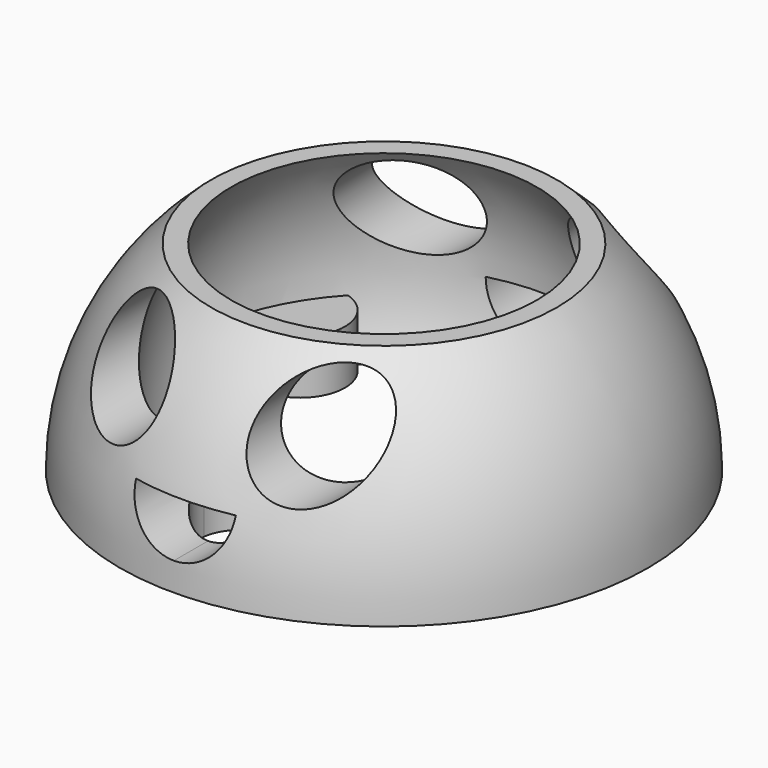
from build123d import *

# Parameters (mm, degrees)
F3_R          = 5.715
F3_R_2        = 5.08
F4_DEPTH      = 6.858
F5_DEPTH      = 6.35
F6_R          = 6.35
F7_DEPTH      = 34.4242277888
F7_DEPTH_BACK = 34.4242277888


# Not quite as in the source:
# - a feature of the source that left no trace in its solid (it failed there, or was rolled back) is left out


with BuildPart() as f1:
    # F0 (on Front) → F1 (revolve)
    with BuildSketch(Plane.XZ):
        with BuildLine():
            ThreePointArc((-22.0018694124, 25.4), (-30.5663007064, 13.9622175447), (-33.6042, 0))
            Line((-33.6042, 0), (-22.9108, 0))
            ThreePointArc((-22.9108, 0), (-24.701230299, 13.1772689339), (-19.4618694124, 25.4))
            Line((-19.4618694124, 25.4), (-22.0018694124, 25.4))
        make_face()
        with BuildLine():
            ThreePointArc((19.4618694124, 25.4), (24.701230299, 13.1772689339), (22.9108, 0))
            Line((22.9108, 0), (33.6042, 0))
            ThreePointArc((33.6042, 0), (30.5663007064, 13.9622175447), (22.0018694124, 25.4))
            Line((22.0018694124, 25.4), (19.4618694124, 25.4))
        make_face()
    revolve(axis=Axis((0, 0, 12.7), (0, 0, 1)))

    # F3 (on face) → F4 (join)
    with BuildSketch(Plane(origin=(0, 0, 0), x_dir=(1, 0, 0), z_dir=(0, 0, -1))):
        with Locations((0, 22.9108)):
            Circle(F3_R)
        with Locations((0, 22.9108)):
            Circle(F3_R_2, mode=Mode.SUBTRACT)
        with Locations((-19.841334821, -11.4554)):
            Circle(F3_R)
        with Locations((-19.841334821, -11.4554)):
            Circle(F3_R_2, mode=Mode.SUBTRACT)
        with Locations((19.841334821, -11.4554)):
            Circle(F3_R)
        with Locations((19.841334821, -11.4554)):
            Circle(F3_R_2, mode=Mode.SUBTRACT)
        with BuildLine():
            ThreePointArc((-16.8292532791, -15.5460924579), (-19.841334821, -11.4554), (-21.8779376376, -6.8015146375))
            ThreePointArc((-21.8779376376, -6.8015146375), (-24.2407438722, -13.9954), (-16.8292532791, -15.5460924579))
        make_face()
        with BuildLine():
            ThreePointArc((-14.761334821, -11.4554), (-17.0610059114, -7.2037919331), (-21.8779376376, -6.8015146375))
            ThreePointArc((-21.8779376376, -6.8015146375), (-19.841334821, -11.4554), (-16.8292532791, -15.5460924579))
            ThreePointArc((-16.8292532791, -15.5460924579), (-15.307695321, -13.747236138), (-14.761334821, -11.4554))
        make_face()
        with BuildLine():
            ThreePointArc((16.8292532791, -15.5460924579), (19.841334821, -11.4554), (21.8779376376, -6.8015146375))
            ThreePointArc((21.8779376376, -6.8015146375), (15.4419257698, -8.9154), (16.8292532791, -15.5460924579))
        make_face()
        with BuildLine():
            ThreePointArc((24.921334821, -11.4554), (24.0929428879, -8.6750710904), (21.8779376376, -6.8015146375))
            ThreePointArc((21.8779376376, -6.8015146375), (19.841334821, -11.4554), (16.8292532791, -15.5460924579))
            ThreePointArc((16.8292532791, -15.5460924579), (22.133170959, -15.9890395001), (24.921334821, -11.4554))
        make_face()
        with BuildLine():
            ThreePointArc((5.0486843585, 22.3476070953), (0, 22.9108), (-5.0486843585, 22.3476070953))
            ThreePointArc((-5.0486843585, 22.3476070953), (0, 17.8308), (5.0486843585, 22.3476070953))
        make_face()
        with BuildLine():
            ThreePointArc((5.08, 22.9108), (-0.2820314332, 27.9829650477), (-5.0486843585, 22.3476070953))
            ThreePointArc((-5.0486843585, 22.3476070953), (0, 22.9108), (5.0486843585, 22.3476070953))
            ThreePointArc((5.0486843585, 22.3476070953), (5.0721650477, 22.6287685668), (5.08, 22.9108))
        make_face()
    extrude(amount=-F4_DEPTH)

    # F3 (on face) → F5 (cut)
    with BuildSketch(Plane(origin=(0, 0, 0), x_dir=(1, 0, 0), z_dir=(0, 0, -1))):
        with BuildLine():
            ThreePointArc((-14.761334821, -11.4554), (-17.0610059114, -7.2037919331), (-21.8779376376, -6.8015146375))
            ThreePointArc((-21.8779376376, -6.8015146375), (-19.841334821, -11.4554), (-16.8292532791, -15.5460924579))
            ThreePointArc((-16.8292532791, -15.5460924579), (-15.307695321, -13.747236138), (-14.761334821, -11.4554))
        make_face()
        with BuildLine():
            ThreePointArc((-16.8292532791, -15.5460924579), (-19.841334821, -11.4554), (-21.8779376376, -6.8015146375))
            ThreePointArc((-21.8779376376, -6.8015146375), (-24.2407438722, -13.9954), (-16.8292532791, -15.5460924579))
        make_face()
        with BuildLine():
            ThreePointArc((5.0486843585, 22.3476070953), (0, 22.9108), (-5.0486843585, 22.3476070953))
            ThreePointArc((-5.0486843585, 22.3476070953), (0, 17.8308), (5.0486843585, 22.3476070953))
        make_face()
        with BuildLine():
            ThreePointArc((5.08, 22.9108), (-0.2820314332, 27.9829650477), (-5.0486843585, 22.3476070953))
            ThreePointArc((-5.0486843585, 22.3476070953), (0, 22.9108), (5.0486843585, 22.3476070953))
            ThreePointArc((5.0486843585, 22.3476070953), (5.0721650477, 22.6287685668), (5.08, 22.9108))
        make_face()
        with BuildLine():
            ThreePointArc((16.8292532791, -15.5460924579), (19.841334821, -11.4554), (21.8779376376, -6.8015146375))
            ThreePointArc((21.8779376376, -6.8015146375), (15.4419257698, -8.9154), (16.8292532791, -15.5460924579))
        make_face()
        with BuildLine():
            ThreePointArc((24.921334821, -11.4554), (24.0929428879, -8.6750710904), (21.8779376376, -6.8015146375))
            ThreePointArc((21.8779376376, -6.8015146375), (19.841334821, -11.4554), (16.8292532791, -15.5460924579))
            ThreePointArc((16.8292532791, -15.5460924579), (22.133170959, -15.9890395001), (24.921334821, -11.4554))
        make_face()
    extrude(amount=-F5_DEPTH, mode=Mode.SUBTRACT)

    # F6 (on Front) → F7 (cut, two sides)
    with BuildSketch(Plane.XZ) as f7_sk:
        with BuildLine():
            Line((6.35, 9.8232205588), (0, 9.8232205588))
            Line((0, 9.8232205588), (0, 3.4732205588))
            ThreePointArc((0, 3.4732205588), (4.4901280605, 5.3330924982), (6.35, 9.8232205588))
        make_face()
        with BuildLine():
            Line((0, 3.4732205588), (0, 9.8232205588))
            Line((0, 9.8232205588), (-6.35, 9.8232205588))
            ThreePointArc((-6.35, 9.8232205588), (-4.4901280605, 5.3330924982), (0, 3.4732205588))
        make_face()
        with BuildLine():
            ThreePointArc((-18.1619651171, 17.78), (-11.8119651171, 11.43), (-5.4619651171, 17.78))
            Line((-5.4619651171, 17.78), (-18.1619651171, 17.78))
        make_face()
        with BuildLine():
            Line((-18.1619651171, 17.78), (-5.4619651171, 17.78))
            ThreePointArc((-5.4619651171, 17.78), (-11.8119651171, 24.13), (-18.1619651171, 17.78))
        make_face()
        with Locations((11.8119651171, 17.78)):
            Circle(F6_R)
    extrude(amount=F7_DEPTH, mode=Mode.SUBTRACT)
    extrude(f7_sk.sketch, amount=-F7_DEPTH_BACK, mode=Mode.SUBTRACT)


solid = f1.part
